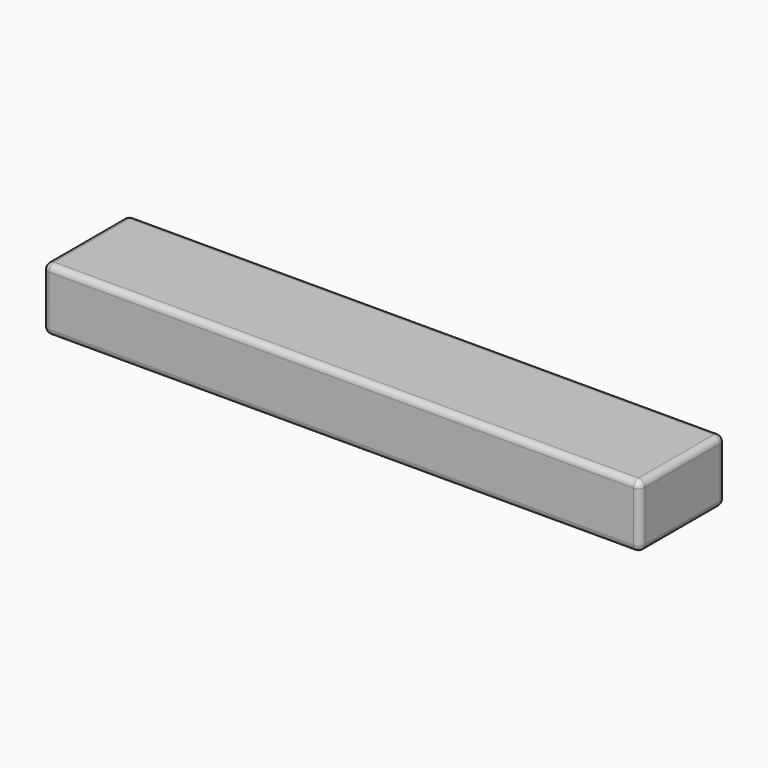
from build123d import *

# Parameters (mm, degrees)
F0_W     = 95
F0_H     = 17
F1_DEPTH = 10
F2_T     = -3
F3_R     = 1


with BuildPart() as f1:
    # F0 (on Top) → F1 (new body)
    with BuildSketch(Plane.XY):
        with Locations((-0.1398691535, -5.5)):
            Rectangle(F0_W, F0_H)
    extrude(amount=F1_DEPTH)

    # F2
    f2_openings = [f1.faces().sort_by_distance(p)[0] for p in [
        (-0.139869, -5.5, 0),
    ]]
    offset(amount=F2_T, openings=f2_openings)

    # F3
    f3_edges = [f1.edges().sort_by_distance(p)[0] for p in [
        (-44.639869, -5.5, 7),
        (-0.139869, -11, 7),
        (44.360131, -5.5, 7),
        (-0.139869, 0, 7),
        (-0.139869, 0, 0),
        (44.360131, 0, 3.5),
        (-44.639869, 0, 3.5),
        (-0.139869, -11, 0),
        (-44.639869, -11, 3.5),
        (44.360131, -11, 3.5),
        (47.360131, -14, 5),
        (47.360131, 3, 5),
        (47.360131, -5.5, 0),
        (47.360131, -5.5, 10),
        (-47.639869, -14, 5),
        (-0.139869, -14, 0),
        (-0.139869, -14, 10),
        (-47.639869, 3, 5),
        (-0.139869, 3, 0),
        (-0.139869, 3, 10),
        (-47.639869, -5.5, 0),
        (-47.639869, -5.5, 10),
        (44.360131, -5.5, 0),
        (-44.639869, -5.5, 0),
    ]]
    fillet(f3_edges, radius=F3_R)


solid = f1.part
